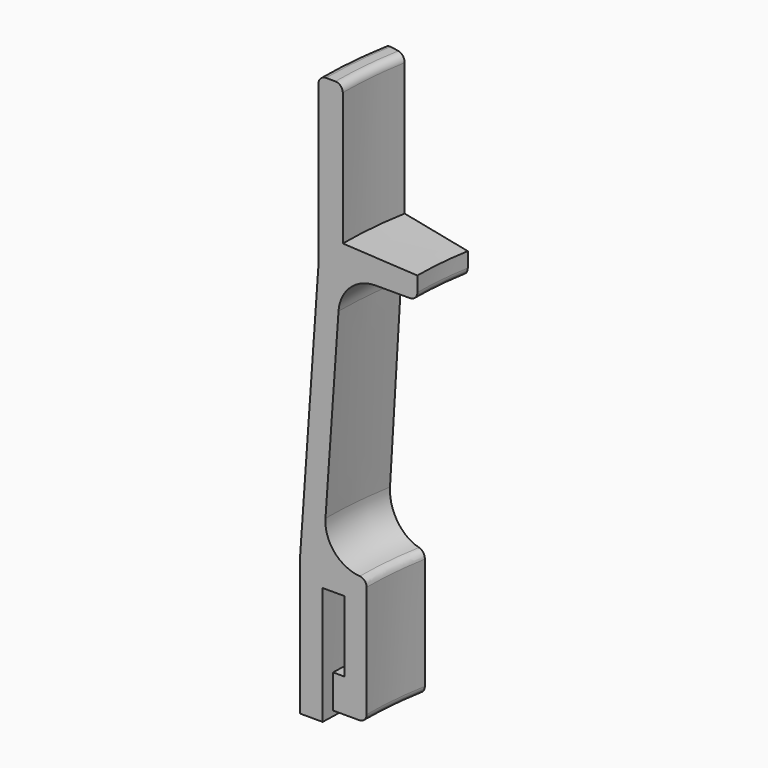
from build123d import *

# Parameters (mm, degrees)
F1_ANGLE = 10
F2_R     = 5
F3_R     = 1


# Not quite as in the source:
# - a feature names something its author has since deleted; it is built from what else it names


with BuildPart() as f1:
    # F0 (on Front) → F1 (revolve)
    with BuildSketch(Plane.XZ):
        Polygon((-3, 0), (0, 0), (0, 15.8), (2.9, 15.8), (2.9, 6.3), (1.4, 6.3), (1.4, 1.8), (5.9, 1.8), (5.9, 18.8), (0.0073256942, 18.8), (-3, 18.8), align=None)
        Polygon((-0.552561582, 53.8), (-3, 18.8), (0.0073256942, 18.8), (2.4547641123, 53.8), align=None)
        Polygon((-0.552561582, 76.1240777928), (-0.552561582, 53.8), (2.4547641123, 53.8), (12.7011916374, 53.8), (12.7011916374, 56.8), (2.7011916374, 57.3240777928), (2.7011916374, 76.1240777928), align=None)
    revolve(axis=Axis((56.5, 0, 26.2500001118), (0, 0, -1)), revolution_arc=F1_ANGLE)

    # F2
    f2_edges = [f1.edges().sort_by_distance(p)[0] for p in [
        (0.222297, 4.923661, 18.8),
        (2.660423, 4.710353, 53.8),
    ]]
    fillet(f2_edges, radius=F2_R)

    # F3
    f3_edges = [f1.edges().sort_by_distance(p)[0] for p in [
        (6.092548, 4.410081, 1.8),
        (6.092548, 4.410081, 18.8),
        (12.867859, 3.817318, 53.8),
        (2.905912, 4.688875, 76.124078),
        (-0.335459, 4.972458, 76.124078),
    ]]
    fillet(f3_edges, radius=F3_R)


solid = f1.part
